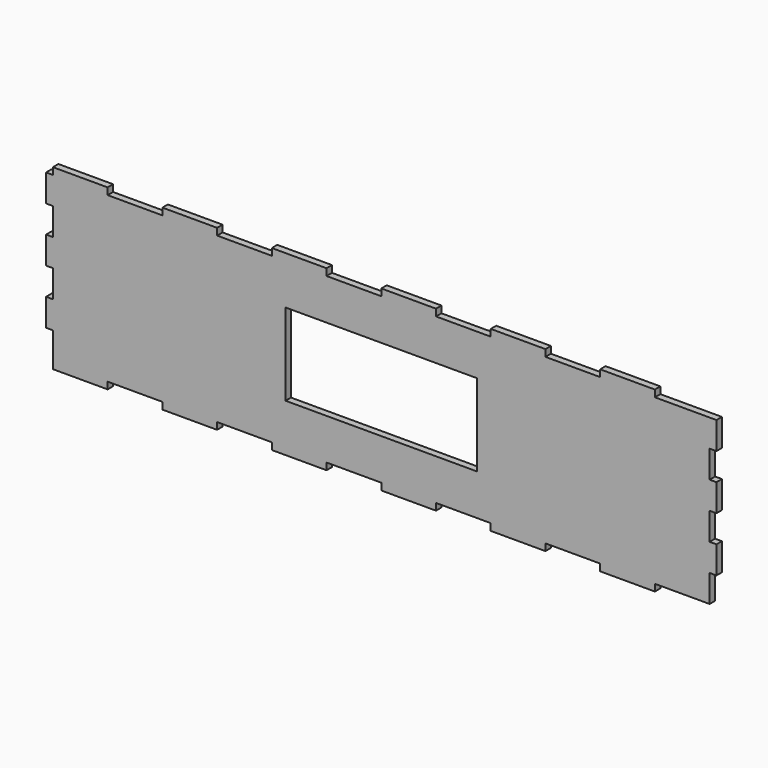
from build123d import *

# Parameters (mm, degrees)
F1_DEPTH = 3.175
F2_W     = 88.9
F2_H     = 38.1
F3_DEPTH = 25.4


# Not quite as in the source:
# - a length typed as a fraction of an inch, garbled in the dataset ("3 / 203.2 mm" for 3/8 in), is restored


with BuildPart() as f1:
    # F0 (on Front) → F1 (new body)
    with BuildSketch(Plane.XZ):
        Polygon((50.8, 0), (25.4, 0), (25.4, 3.175), (0, 3.175), (0, 0), (-3.175, 0), (-3.175, -12.7), (0, -12.7), (0, -25.4), (-3.175, -25.4), (-3.175, -38.1), (0, -38.1), (0, -50.8), (-3.175, -50.8), (-3.175, -63.5), (0, -63.5), (0, -76.2), (0, -79.375), (25.4, -79.375), (25.4, -76.2), (50.8, -76.2), (50.8, -79.375), (76.2, -79.375), (76.2, -76.2), (101.6, -76.2), (101.6, -79.375), (127, -79.375), (127, -76.2), (152.4, -76.2), (152.4, -79.375), (177.8, -79.375), (177.8, -76.2), (203.2, -76.2), (203.2, -79.375), (228.6, -79.375), (228.6, -76.2), (254, -76.2), (254, -79.375), (279.4, -79.375), (279.4, -76.2), (304.8, -76.2), (304.8, -63.5), (307.975, -63.5), (307.975, -50.8), (304.8, -50.8), (304.8, -38.1), (307.975, -38.1), (307.975, -25.4), (304.8, -25.4), (304.8, -12.7), (307.975, -12.7), (307.975, 0), (304.8, 0), (279.4, 0), (279.4, 3.175), (254, 3.175), (254, 0), (228.6, 0), (228.6, 3.175), (203.2, 3.175), (203.2, 0), (177.8, 0), (177.8, 3.175), (152.4, 3.175), (152.4, 0), (127, 0), (127, 3.175), (101.6, 3.175), (101.6, 0), (76.2, 0), (76.2, 3.175), (50.8, 3.175), align=None)
    extrude(amount=F1_DEPTH)

    # F2 (on face) → F3 (cut)
    with BuildSketch(Plane.XZ.offset(3.175)):
        with Locations((152.4, -38.1)):
            Rectangle(F2_W, F2_H)
    extrude(amount=-F3_DEPTH, mode=Mode.SUBTRACT)


solid = f1.part
